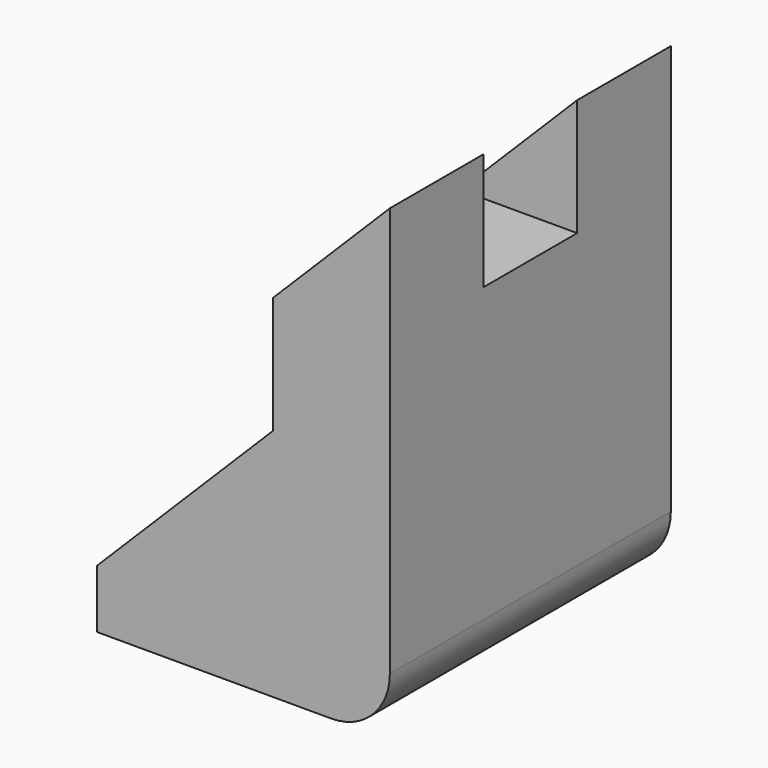
from build123d import *

# Parameters (mm, degrees)
F5_W        = 10
F5_H        = 10
F0_DEPTH    = 30
F1_DEPTH    = 10
F7_DEPTH    = 10
F3_D        = 5
F3_DEPTH    = 15
F3_TIP      = 1.5021515476
F8_D        = 5
F8_DEPTH    = 5
F8_TIP      = 1.5021515476
F4_T1_DEPTH = 55


# Not quite as in the source:
# - a fillet or chamfer that OpenCascade refuses, or shapes differently, is made with other operations: its cross-section is extruded or revolved along the edge and cut away or added


with BuildPart() as f0:
    # F5 (on Front) → F0 (new body)
    with BuildSketch(Plane.XZ):
        Polygon((10, 20), (10, 10), (20, 20), align=None)
        Polygon((20, 20), (10, 10), (20, 10), align=None)
        with Locations((15, 5)):
            Rectangle(F5_W, F5_H)
        Polygon((10, 10), (0, 0), (10, 0), align=None)
        Polygon((10, 0), (0, 0), (-5, -5), (-5, -10), (20, -10), (20, 0), align=None)
    extrude(amount=F0_DEPTH)

    # F5 (on Front) → F1 (join)
    with BuildSketch(Plane.XZ):
        Polygon((10, 20), (20, 20), (20, 30), align=None)
    extrude(amount=F1_DEPTH)

    # F6 (on face) → F7 (join)
    with BuildSketch(Plane.XZ.offset(30)):
        Polygon((10, 20), (20, 20), (20, 30), align=None)
    extrude(amount=-F7_DEPTH)

    # F3
    with Locations(Plane(origin=(0, 0, -10), x_dir=(1, 0, 0), z_dir=(0, 0, -1))):
        with Locations((15, 15)):
            Hole(F3_D / 2, depth=F3_DEPTH)
            with Locations((0, 0, -(F3_DEPTH + F3_TIP / 2))):  # 118° drill point
                Cone(0, F3_D / 2, F3_TIP, mode=Mode.SUBTRACT)

    # F8
    with Locations(Plane(origin=(0, 0, -10), x_dir=(1, 0, 0), z_dir=(0, 0, -1))):
        with Locations((7.5, 15), (0, 15)):
            Hole(F8_D / 2, depth=F8_DEPTH)
            with Locations((0, 0, -(F8_DEPTH + F8_TIP / 2))):  # 118° drill point
                Cone(0, F8_D / 2, F8_TIP, mode=Mode.SUBTRACT)

    # F4: fillet of radius 5 on 1 edges, made by hand

    # F4_s2 → F4_t1 (cut)
    with BuildSketch(Plane.XZ.offset(-12.5)):
        with BuildLine():
            ThreePointArc((20, -5), (18.5355339059, -8.5355339059), (15, -10))
            Line((15, -10), (20, -10))
            Line((20, -10), (20, -5))
        make_face()
    extrude(amount=F4_T1_DEPTH, mode=Mode.SUBTRACT)


solid = f0.part
